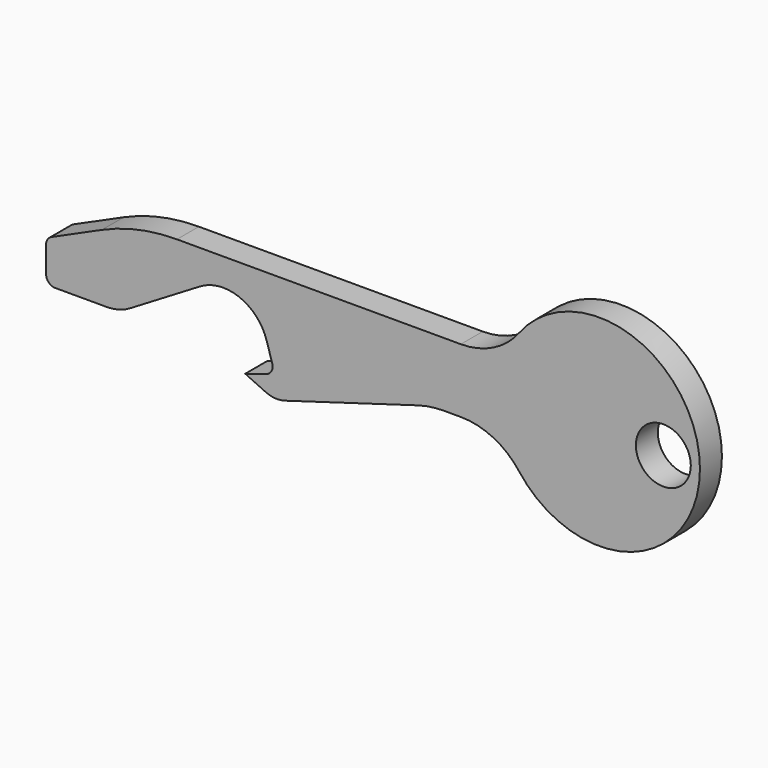
from build123d import *

# Parameters (mm, degrees)
F0_R        = 3
F1_DEPTH    = 3
F2_R        = 10
F3_R        = 5
F4_R        = 1
F5_T1_DEPTH = 3
F6_R        = 20
F7_R        = 1
F8_R        = 3
F9_R        = 8


# Not quite as in the source:
# - a fillet or chamfer that OpenCascade refuses, or shapes differently, is made with other operations: its cross-section is extruded or revolved along the edge and cut away or added
# - a feature names something its author has since deleted; it is built from what else it names


with BuildPart() as f1:
    # F0 (on Front) → F1 (new body)
    with BuildSketch(Plane.XZ):
        Polygon((-2, -2), (1.3333333333, 0), (0, 0), (0, 7), (-10, 2.5), (-10, -2), align=None)
        Polygon((14.2307692308, 0), (32, 0), (40, 0), (40, 7), (0, 7), (0, 0), (1.3333333333, 0), (8, 4), (13, 4), align=None)
        Polygon((15, -5), (32, 0), (14.2307692308, 0), (15, -2.5), (11.75, -3.5), align=None)
        with BuildLine():
            Line((40, 7), (40, 0))
            ThreePointArc((40, 0), (61.4283268073, 3.5), (40, 7))
        make_face()
        with Locations((57.4283268073, 3.5)):
            Circle(F0_R, mode=Mode.SUBTRACT)
    extrude(amount=F1_DEPTH)

    # F2
    f2_edges = [f1.edges().sort_by_distance(p)[0] for p in [
        (32, -1.5, 0),
    ]]
    fillet(f2_edges, radius=F2_R)

    # F3
    f3_edges = [f1.edges().sort_by_distance(p)[0] for p in [
        (13, -1.5, 4),
        (-2, -1.5, -2),
    ]]
    fillet(f3_edges, radius=F3_R)

    # F4
    f4_edges = [f1.edges().sort_by_distance(p)[0] for p in [
        (15, -1.5, -2.5),
    ]]
    fillet(f4_edges, radius=F4_R)

    # F5: fillet of radius 5 on 1 edges, made by hand

    # F5_s2 → F5_t1 (join)
    with BuildSketch(Plane.XZ):
        with BuildLine():
            ThreePointArc((9.3849198247, 4), (8.0502519153, 3.8185746411), (6.8124410476, 3.2874646286))
            Line((6.8124410476, 3.2874646286), (8, 4))
            Line((8, 4), (9.3849198247, 4))
        make_face()
    extrude(amount=F5_T1_DEPTH)

    # F6
    f6_edges = [f1.edges().sort_by_distance(p)[0] for p in [
        (0, -1.5, 7),
    ]]
    fillet(f6_edges, radius=F6_R)

    # F7
    f7_edges = [f1.edges().sort_by_distance(p)[0] for p in [
        (-10, -1.5, 2.5),
        (-10, -1.5, -2),
    ]]
    fillet(f7_edges, radius=F7_R)

    # F8
    f8_edges = [f1.edges().sort_by_distance(p)[0] for p in [
        (15, -1.5, -5),
    ]]
    fillet(f8_edges, radius=F8_R)

    # F9
    f9_edges = [f1.edges().sort_by_distance(p)[0] for p in [
        (40, -1.5, 7),
        (40, -1.5, 0),
    ]]
    fillet(f9_edges, radius=F9_R)


solid = f1.part
